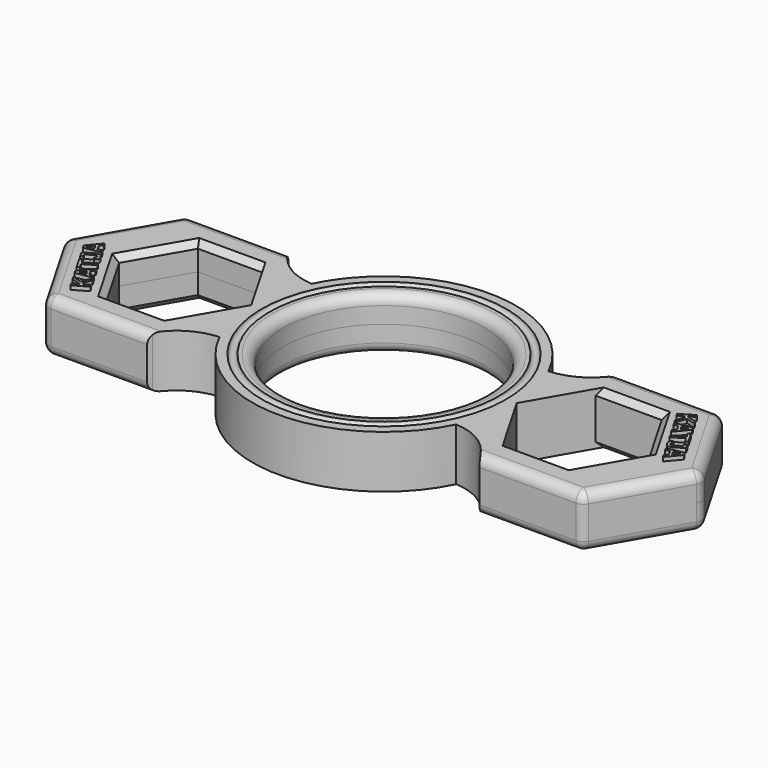
from build123d import *

# Parameters (mm, degrees)
F0_R     = 15.35
F1_DEPTH = 4
F2_R     = 1.5
F3_SIZE  = 0.9
F5_DEPTH = 0.6
F6_R     = 0.6


# Not quite as in the source:
# - a feature names something its author has since deleted; it is built from what else it names


with BuildPart() as f1:
    # F0 (on Top) → F1 (new body, symmetric)
    with BuildSketch(Plane.XY):
        with BuildLine():
            Line((-25.2499836894, -13.4233655079), (-24.9054608768, -12.8266344921))
            ThreePointArc((-24.9054608768, -12.8266344921), (-25.0835939354, -13.12161), (-25.2499836894, -13.4233655079))
        make_face()
        with BuildLine():
            ThreePointArc((-25.2499863666, 13.4233648625), (-25.0835962475, 13.1216086651), (-24.9054627744, 12.8266324963))
            Line((-24.9054627744, 12.8266324963), (-25.2499863666, 13.4233648625))
        make_face()
        with BuildLine():
            Line((25.2499979173, 13.4233925562), (24.9054452913, 12.8266097953))
            ThreePointArc((24.9054452913, 12.8266097953), (25.083594275, 13.1216105883), (25.2499979173, 13.4233925562))
        make_face()
        with BuildLine():
            ThreePointArc((25.25, -13.4233937587), (25.0835950469, -13.1216093583), (24.9054445662, -12.8266062413))
            Line((24.9054445662, -12.8266062413), (25.25, -13.4233937587))
        make_face()
        with BuildLine():
            ThreePointArc((-14.9303856554, -9.1287230312), (-16.4393462193, -8.8076925085), (-17.9812272394, -8.7564528758))
            ThreePointArc((-17.9812272394, -8.7564528758), (6.962e-07, -20), (17.981227849, -8.756451624))
            ThreePointArc((17.981227849, -8.756451624), (16.439347052, -8.8076911139), (14.930386666, -9.1287213784))
            ThreePointArc((14.930386666, -9.1287213784), (9.686e-07, -17.5), (-14.9303856554, -9.1287230312))
        make_face()
        with BuildLine():
            ThreePointArc((-14.9303877575, 9.1287195931), (-2.0149e-06, 17.5), (14.9303856554, 9.1287230312))
            ThreePointArc((14.9303856554, 9.1287230312), (16.4393462193, 8.8076925085), (17.9812272394, 8.7564528758))
            ThreePointArc((17.9812272394, 8.7564528758), (2.4245927758, 19.8524897651), (-15.3452761072, 12.8266324963))
            ThreePointArc((-15.3452761072, 12.8266324963), (-16.7870656546, 10.8717260224), (-17.9812285075, 8.7564502717))
            ThreePointArc((-17.9812285075, 8.7564502717), (-16.4393479515, 8.8076896075), (-14.9303877575, 9.1287195931))
        make_face()
        with BuildLine():
            ThreePointArc((24.9054452913, 12.8266097953), (21.9375043931, 9.9508443698), (17.9812272394, 8.7564528758))
            ThreePointArc((17.9812272394, 8.7564528758), (19.4887729833, 4.4930755176), (20, 0))
            ThreePointArc((20, 0), (19.4887731397, -4.4930748391), (17.981227849, -8.756451624))
            ThreePointArc((17.981227849, -8.756451624), (21.9375038139, -9.9508425405), (24.9054445662, -12.8266062413))
            ThreePointArc((24.9054445662, -12.8266062413), (25.0835950469, -13.1216093583), (25.25, -13.4233937587))
            Line((25.25, -13.4233937587), (40.75, -13.4233937587))
            Line((40.75, -13.4233937587), (48.5, 0))
            Line((48.5, 0), (40.75, 13.4233937587))
            Line((40.75, 13.4233937587), (25.2499979173, 13.4233925562))
            ThreePointArc((25.2499979173, 13.4233925562), (25.083594275, 13.1216105883), (24.9054452913, 12.8266097953))
        make_face()
        Polygon((25.1845580846, -8.703555308), (20.1595580846, 0), (25.1845580846, 8.703555308), (35.2345580846, 8.703555308), (40.2595580846, 0), (35.2345580846, -8.703555308), align=None, mode=Mode.SUBTRACT)
        with BuildLine():
            ThreePointArc((17.9812272394, 8.7564528758), (16.4393462193, 8.8076925085), (14.9303856554, 9.1287230312))
            ThreePointArc((14.9303856554, 9.1287230312), (-2.0149e-06, 17.5), (-14.9303877575, 9.1287195931))
            ThreePointArc((-14.9303877575, 9.1287195931), (-16.4393479515, 8.8076896075), (-17.9812285075, 8.7564502717))
            ThreePointArc((-17.9812285075, 8.7564502717), (-20, -1.4482e-06), (-17.9812272394, -8.7564528758))
            ThreePointArc((-17.9812272394, -8.7564528758), (-16.4393462193, -8.8076925085), (-14.9303856554, -9.1287230312))
            ThreePointArc((-14.9303856554, -9.1287230312), (9.686e-07, -17.5), (14.930386666, -9.1287213784))
            ThreePointArc((14.930386666, -9.1287213784), (16.439347052, -8.8076911139), (17.981227849, -8.756451624))
            ThreePointArc((17.981227849, -8.756451624), (19.4887731397, -4.4930748391), (20, 0))
            ThreePointArc((20, 0), (19.4887729833, 4.4930755176), (17.9812272394, 8.7564528758))
        make_face()
        Circle(F0_R, mode=Mode.SUBTRACT)
        with BuildLine():
            ThreePointArc((-17.9812272394, -8.7564528758), (-20, -1.4482e-06), (-17.9812285075, 8.7564502717))
            ThreePointArc((-17.9812285075, 8.7564502717), (-21.9375185272, 9.950849581), (-24.9054627744, 12.8266324963))
            ThreePointArc((-24.9054627744, 12.8266324963), (-25.0835962475, 13.1216086651), (-25.2499863666, 13.4233648625))
            Line((-25.2499863666, 13.4233648625), (-40.7499537455, 13.4233648625))
            Line((-40.7499537455, 13.4233648625), (-48.4999374349, -6.454e-07))
            Line((-48.4999374349, -6.454e-07), (-40.7499537455, -13.4233661533))
            Line((-40.7499537455, -13.4233661533), (-25.2499836894, -13.4233655079))
            ThreePointArc((-25.2499836894, -13.4233655079), (-25.0835939354, -13.12161), (-24.9054608768, -12.8266344921))
            ThreePointArc((-24.9054608768, -12.8266344921), (-21.9375169811, -9.9508517692), (-17.9812272394, -8.7564528758))
        make_face()
        Polygon((-25.1845580846, 8.703555308), (-20.1595580846, 0), (-25.1845580846, -8.703555308), (-35.2345580846, -8.703555308), (-40.2595580846, 0), (-35.2345580846, 8.703555308), align=None, mode=Mode.SUBTRACT)
    extrude(amount=F1_DEPTH, both=True)

    # F2
    f2_edges = [f1.edges().sort_by_distance(p)[0] for p in [
        (44.625, 6.711697, -4),
        (40.75, 13.423394, 0),
        (44.625, 6.711697, 4),
        (48.5, 0, 0),
        (32.999999, 13.423393, -4),
        (32.999999, 13.423393, 4),
        (33, -13.423394, 4),
        (44.625, -6.711697, 4),
        (40.75, -13.423394, 0),
        (44.625, -6.711697, -4),
        (33, -13.423394, -4),
        (-32.999969, -13.423366, -4),
        (-44.624946, -6.711683, -4),
        (-44.624946, 6.711682, -4),
        (-32.99997, 13.423365, -4),
        (-44.624946, 6.711682, 4),
        (-48.499937, -1e-06, 0),
        (-44.624946, -6.711683, 4),
        (-32.999969, -13.423366, 4),
        (-40.749954, -13.423366, 0),
        (-40.749954, 13.423365, 0),
        (-32.99997, 13.423365, 4),
        (-15.35, 0, 4),
        (-15.35, 0, -4),
    ]]
    fillet(f2_edges, radius=F2_R)

    # F3
    f3_edges = [f1.edges().sort_by_distance(p)[0] for p in [
        (30.209558, 8.703555, 4),
        (30.209558, 8.703555, -4),
        (37.747058, 4.351778, -4),
        (37.747058, 4.351778, 4),
        (37.747058, -4.351778, 4),
        (37.747058, -4.351778, -4),
        (30.209558, -8.703555, 4),
        (-30.209558, 8.703555, 4),
        (-37.747058, 4.351778, 4),
        (-37.747058, -4.351778, 4),
        (-30.209558, -8.703555, 4),
        (30.209558, -8.703555, -4),
        (-37.747058, 4.351778, -4),
        (-37.747058, -4.351778, -4),
        (-30.209558, -8.703555, -4),
        (-30.209558, 8.703555, -4),
    ]]
    chamfer(f3_edges, length=F3_SIZE)

    # F4 (on face) → F5 (join)
    with BuildSketch(Plane.XY.offset(4)):
        Polygon((39.5191783421, 10.0599360948), (37.4504338473, 8.8655459038), (37.7005423542, 8.4323452624), (38.4551196103, 8.8680006444), (38.7981461772, 8.7252500912), (38.2769854966, 7.4339164522), (38.5721243855, 6.9227209013), (39.2139812382, 8.5681536795), (40.5990937067, 8.1894678155), (40.3074812935, 8.6945553313), (38.8309986918, 9.0850145332), (39.769286849, 9.6267354534), align=None)
        Polygon((44.4155542101, 1.5791643184), (41.910883066, 1.1398212324), (42.160991573, 0.706620591), (42.7956370695, 0.8280854711), (43.2508237015, 0.0396790977), (42.8283092813, -0.4492075847), (43.0757051146, -0.8777097376), (44.7104218317, 1.0684386164), align=None)
        with BuildLine():
            Line((43.9973752238, 0.8722649721), (43.5210177283, 0.3247275098))
            Line((43.5210177283, 0.3247275098), (43.1775932491, 0.9195561562))
            add(Edge.make_bspline(
                [(44.0662304905, 1.0958860963), (43.9867721257, 1.0772620213), (43.1775932491, 0.9195561562)],
                knots=[0, 0, 0, 1, 1, 1], degree=2))
            add(Edge.make_bspline(
                [(44.2442948657, 1.140117121), (44.1456888554, 1.1145101712), (44.0662304905, 1.0958860963)],
                knots=[0, 0, 0, 1, 1, 1], degree=2))
            Line((44.2442948657, 1.140117121), (43.9973752238, 0.8722649721))
        make_face(mode=Mode.SUBTRACT)
        with BuildLine():
            add(Edge.make_bspline(
                [(41.193782065, 2.3818766002), (41.1496463709, 2.5383871398), (41.1712183224, 2.674864399)],
                knots=[0.4605661865, 0.4605661865, 0.4605661865, 1, 1, 1], degree=2))
            Line((41.193782065, 2.3818766002), (41.4871422415, 1.8737618696))
            add(Edge.make_bspline(
                [(41.7943342202, 1.6905395814), (41.6237528486, 1.7376651114), (41.4871422415, 1.8737618696)],
                knots=[0, 0, 0, 0.5952171511, 0.5952171511, 0.5952171511], degree=2))
            add(Edge.make_bspline(
                [(42.4041770183, 1.7979978495), (42.0809210082, 1.6113659051), (41.7943342202, 1.6905395814)],
                knots=[0, 0, 0, 1, 1, 1], degree=2))
            Line((42.4041770183, 1.7979978495), (43.8179522136, 2.6142413391))
            Line((43.8179522136, 2.6142413391), (43.3304847657, 3.4585597259))
            Line((43.3304847657, 3.4585597259), (42.9912538946, 3.2627046912))
            Line((42.9912538946, 3.2627046912), (43.2294266377, 2.8501773992))
            Line((43.2294266377, 2.8501773992), (42.1445456387, 2.2238210624))
            add(Edge.make_bspline(
                [(41.8577105552, 2.1471747991), (41.9829176337, 2.1305050902), (42.1445456387, 2.2238210624)],
                knots=[0, 0, 0, 1, 1, 1], degree=2))
            add(Edge.make_bspline(
                [(41.6579049525, 2.2930529422), (41.7325034768, 2.1638445079), (41.8577105552, 2.1471747991)],
                knots=[0, 0, 0, 1, 1, 1], degree=2))
            add(Edge.make_bspline(
                [(41.6207202622, 2.5359526386), (41.5849340323, 2.4194422833), (41.6579049525, 2.2930529422)],
                knots=[0, 0, 0, 1, 1, 1], degree=2))
            add(Edge.make_bspline(
                [(41.8010641295, 2.7710054323), (41.6565064921, 2.6524629938), (41.6207202622, 2.5359526386)],
                knots=[0, 0, 0, 1, 1, 1], degree=2))
            Line((41.8010641295, 2.7710054323), (41.4896234806, 3.1650371542))
            add(Edge.make_bspline(
                [(41.1712183224, 2.674864399), (41.2112083098, 2.9278653339), (41.4896234806, 3.1650371542)],
                knots=[0, 0, 0, 1, 1, 1], degree=2))
        make_face()
        with BuildLine():
            Line((41.4871422415, 1.8737618696), (41.193782065, 2.3818766002))
            add(Edge.make_bspline(
                [(41.3170464772, 2.1000170005), (41.231464924, 2.2482485989), (41.193782065, 2.3818766002)],
                knots=[0, 0, 0, 0.4605661865, 0.4605661865, 0.4605661865], degree=2))
            add(Edge.make_bspline(
                [(41.4871422415, 1.8737618696), (41.394238953, 1.9663157105), (41.3170464772, 2.1000170005)],
                knots=[0.5952171511, 0.5952171511, 0.5952171511, 1, 1, 1], degree=2))
        make_face()
        Polygon((41.9814124526, 5.0226520708), (40.2472003403, 4.021404241), (40.4973088473, 3.5882035995), (42.2315209596, 4.5894514294), (42.6180769491, 3.9199168155), (42.9526093317, 4.1130591766), (41.9302026476, 5.8839194993), (41.5956702651, 5.6907771382), align=None)
        Polygon((41.1359318143, 7.2596369376), (38.6312606702, 6.8202938516), (38.8813691771, 6.3870932102), (39.5160146737, 6.5085580903), (39.9712013056, 5.7201517169), (39.5486868855, 5.2312650346), (39.7960827188, 4.8027628816), (41.4307994358, 6.7489112356), align=None)
        with BuildLine():
            Line((40.717752828, 6.5527375914), (40.2413953324, 6.005200129))
            Line((40.2413953324, 6.005200129), (39.8979708533, 6.6000287755))
            add(Edge.make_bspline(
                [(40.7866080947, 6.7763587155), (40.7071497298, 6.7577346406), (39.8979708533, 6.6000287755)],
                knots=[0, 0, 0, 1, 1, 1], degree=2))
            add(Edge.make_bspline(
                [(40.9646724698, 6.8205897402), (40.8660664596, 6.7949827904), (40.7866080947, 6.7763587155)],
                knots=[0, 0, 0, 1, 1, 1], degree=2))
            Line((40.9646724698, 6.8205897402), (40.717752828, 6.5527375914))
        make_face(mode=Mode.SUBTRACT)
        Polygon((-38.1149835851, -7.7145119938), (-38.410122474, -7.203316443), (-39.0519793267, -8.8487492211), (-40.4370917952, -8.4700633571), (-40.145479382, -8.9751508729), (-38.6689967803, -9.3656100749), (-39.6072849375, -9.907330995), (-39.3571764306, -10.3405316365), (-37.2884319358, -9.1461414455), (-37.5385404427, -8.712940804), (-38.2931176988, -9.148596186), (-38.6361442657, -9.0058456328), align=None)
        Polygon((-39.386684974, -5.5118605762), (-39.6340808073, -5.0833584233), (-41.2687975243, -7.0295067773), (-40.9739299028, -7.5402324793), (-38.4692587587, -7.1008893933), (-38.7193672656, -6.6676887518), (-39.3540127622, -6.789153632), (-39.8091993941, -6.0007472585), align=None)
        with BuildLine():
            Line((-40.5557509165, -6.833333133), (-40.079393421, -6.2857956706))
            Line((-40.079393421, -6.2857956706), (-39.7359689418, -6.8806243171))
            add(Edge.make_bspline(
                [(-40.6246061832, -7.0569542571), (-40.5451478183, -7.0383301822), (-39.7359689418, -6.8806243171)],
                knots=[0, 0, 0, 1, 1, 1], degree=2))
            add(Edge.make_bspline(
                [(-40.8026705583, -7.1011852818), (-40.7040645481, -7.0755783321), (-40.6246061832, -7.0569542571)],
                knots=[0, 0, 0, 1, 1, 1], degree=2))
            Line((-40.8026705583, -7.1011852818), (-40.5557509165, -6.833333133))
        make_face(mode=Mode.SUBTRACT)
        Polygon((-40.0851984288, -4.3019997826), (-40.3353069358, -3.8687991412), (-42.0695190481, -4.870046971), (-42.4560750376, -4.2005123571), (-42.7906074202, -4.3936547182), (-41.7682007362, -6.1645150409), (-41.4336683536, -5.9713726798), (-41.8194105411, -5.3032476125), align=None)
        with BuildLine():
            add(Edge.make_bspline(
                [(-41.32514033, -2.1543574113), (-41.2322370415, -2.2469112522), (-41.1550445657, -2.3806125422)],
                knots=[0.5952171511, 0.5952171511, 0.5952171511, 1, 1, 1], degree=2))
            Line((-41.32514033, -2.1543574113), (-41.0317801535, -2.6624721419))
            add(Edge.make_bspline(
                [(-41.1550445657, -2.3806125422), (-41.0694630125, -2.5288441405), (-41.0317801535, -2.6624721419)],
                knots=[0, 0, 0, 0.4605661865, 0.4605661865, 0.4605661865], degree=2))
        make_face()
        with BuildLine():
            Line((-41.0317801535, -2.6624721419), (-41.32514033, -2.1543574113))
            add(Edge.make_bspline(
                [(-41.6323323087, -1.971135123), (-41.4617509371, -2.0182606531), (-41.32514033, -2.1543574113)],
                knots=[0, 0, 0, 0.5952171511, 0.5952171511, 0.5952171511], degree=2))
            add(Edge.make_bspline(
                [(-42.2421751068, -2.0785933911), (-41.9189190967, -1.8919614467), (-41.6323323087, -1.971135123)],
                knots=[0, 0, 0, 1, 1, 1], degree=2))
            Line((-42.2421751068, -2.0785933911), (-43.6559503021, -2.8948368807))
            Line((-43.6559503021, -2.8948368807), (-43.1684828542, -3.7391552675))
            Line((-43.1684828542, -3.7391552675), (-42.8292519832, -3.5433002328))
            Line((-42.8292519832, -3.5433002328), (-43.0674247262, -3.1307729409))
            Line((-43.0674247262, -3.1307729409), (-41.9825437272, -2.5044166041))
            add(Edge.make_bspline(
                [(-41.6957086437, -2.4277703407), (-41.8209157222, -2.4111006318), (-41.9825437272, -2.5044166041)],
                knots=[0, 0, 0, 1, 1, 1], degree=2))
            add(Edge.make_bspline(
                [(-41.495903041, -2.5736484838), (-41.5705015653, -2.4444400495), (-41.6957086437, -2.4277703407)],
                knots=[0, 0, 0, 1, 1, 1], degree=2))
            add(Edge.make_bspline(
                [(-41.4587183507, -2.8165481802), (-41.4229321208, -2.700037825), (-41.495903041, -2.5736484838)],
                knots=[0, 0, 0, 1, 1, 1], degree=2))
            add(Edge.make_bspline(
                [(-41.639062218, -3.0516009739), (-41.4945045806, -2.9330585354), (-41.4587183507, -2.8165481802)],
                knots=[0, 0, 0, 1, 1, 1], degree=2))
            Line((-41.639062218, -3.0516009739), (-41.3276215691, -3.4456326958))
            add(Edge.make_bspline(
                [(-41.0092164109, -2.9554599406), (-41.0492063983, -3.2084608755), (-41.3276215691, -3.4456326958)],
                knots=[0, 0, 0, 1, 1, 1], degree=2))
            add(Edge.make_bspline(
                [(-41.0317801535, -2.6624721419), (-40.9876444594, -2.8189826815), (-41.0092164109, -2.9554599406)],
                knots=[0.4605661865, 0.4605661865, 0.4605661865, 1, 1, 1], degree=2))
        make_face()
        Polygon((-42.6663073698, 0.168612043), (-42.9137032031, 0.5971141959), (-44.5484199202, -1.349034158), (-44.2535522987, -1.85975986), (-41.7488811545, -1.420416774), (-41.9989896615, -0.9872161326), (-42.633635158, -1.1086810128), (-43.08882179, -0.3202746393), align=None)
        with BuildLine():
            Line((-43.8353733123, -1.1528605138), (-43.3590158168, -0.6053230514))
            Line((-43.3590158168, -0.6053230514), (-43.0155913376, -1.2001516979))
            add(Edge.make_bspline(
                [(-43.904228579, -1.3764816379), (-43.8247702142, -1.357857563), (-43.0155913376, -1.2001516979)],
                knots=[0, 0, 0, 1, 1, 1], degree=2))
            add(Edge.make_bspline(
                [(-44.0822929542, -1.4207126626), (-43.9836869439, -1.3951057129), (-43.904228579, -1.3764816379)],
                knots=[0, 0, 0, 1, 1, 1], degree=2))
            Line((-44.0822929542, -1.4207126626), (-43.8353733123, -1.1528605138))
        make_face(mode=Mode.SUBTRACT)
    extrude(amount=F5_DEPTH)

    # F6 (on Right) → F7 (revolve, cut)
    with BuildSketch(Plane.YZ):
        with Locations((17.9876219481, 4)):
            Circle(F6_R)
    revolve(axis=Axis((0, 0, -0.0947553199), (0, 0, -1)), mode=Mode.SUBTRACT)


solid = f1.part
